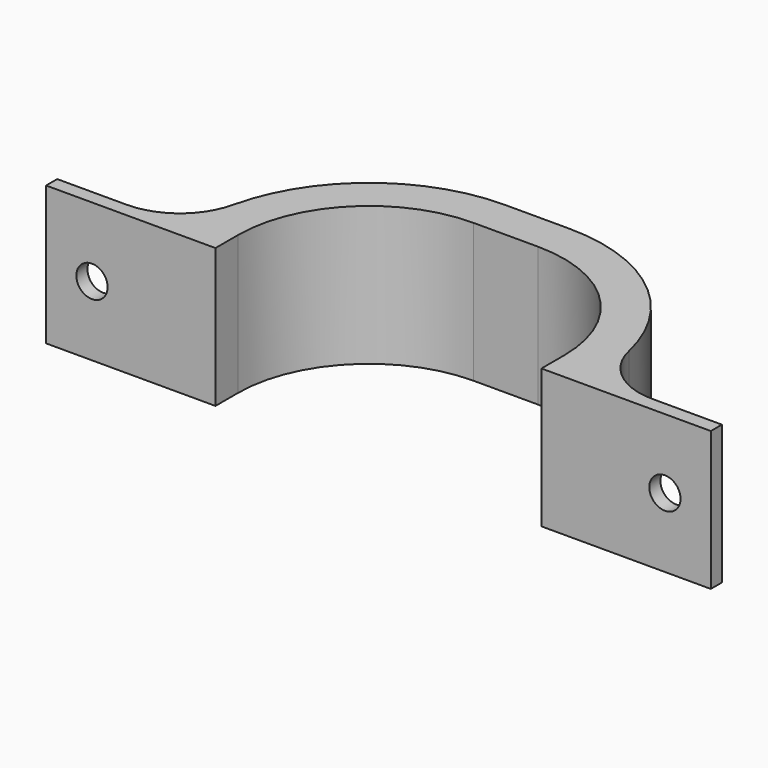
from build123d import *

# Parameters (mm, degrees)
F1_DEPTH = 20
F3_D     = 4.5
F4_D     = 4.5
F5_DEPTH = 2
F6_DEPTH = 2


with BuildPart() as f1:
    # F0 (on Top) → F1 (new body)
    with BuildSketch(Plane.XY):
        with BuildLine():
            Line((-37.8199822518, -7.4723315098), (-45.8199822518, -7.4723315098))
            Line((-45.8199822518, -7.4723315098), (-45.8199822518, -9.4723315098))
            Line((-45.8199822518, -9.4723315098), (-28.8447495745, -9.4723315098))
            Line((-28.8447495745, -9.4723315098), (-23.45, -9.4723315098))
            Line((-23.45, -9.4723315098), (-23.45, -7.887919838))
            Line((-23.45, -7.887919838), (-23.45, -5.3745856304))
            ThreePointArc((-23.45, -5.3745856304), (-17.9429472697, 7.9206157599), (-4.6477458794, 13.4276684902))
            Line((-4.6477458794, 13.4276684902), (0, 13.4276684902))
            Line((0, 13.4276684902), (4.6477458794, 13.4276684902))
            ThreePointArc((4.6477458794, 13.4276684902), (17.9429472697, 7.9206157599), (23.45, -5.3745856304))
            Line((23.45, -5.3745856304), (23.45, -7.887919838))
            Line((23.45, -7.887919838), (23.45, -9.4723315098))
            Line((23.45, -9.4723315098), (28.8447495745, -9.4723315098))
            Line((28.8447495745, -9.4723315098), (45.8199822518, -9.4723315098))
            Line((45.8199822518, -9.4723315098), (45.8199822518, -7.4723315098))
            Line((45.8199822518, -7.4723315098), (37.8199822518, -7.4723315098))
            ThreePointArc((37.8199822518, -7.4723315098), (31.8371692612, -5.3745856304), (28.4743700766, 0))
            ThreePointArc((28.4743700766, 0), (19.9009167747, 13.7024940459), (4.6477458794, 19.0506920822))
            Line((4.6477458794, 19.0506920822), (0, 19.0506920822))
            Line((0, 19.0506920822), (-4.6477458794, 19.0506920822))
            ThreePointArc((-4.6477458794, 19.0506920822), (-19.9009167747, 13.7024940459), (-28.4743700766, 0))
            ThreePointArc((-28.4743700766, 0), (-31.8371692612, -5.3745856304), (-37.8199822518, -7.4723315098))
        make_face()
    extrude(amount=F1_DEPTH)

    # F3 (through all)
    with Locations(Plane(origin=(0, -7.4723315098, 0), x_dir=(-1, 0, 0), z_dir=(0, 1, 0))):
        with Locations((-41.2173499218, 10)):
            Hole(F3_D / 2)

    # F4 (through all)
    with Locations(Plane(origin=(0, -7.4723315098, 0), x_dir=(-1, 0, 0), z_dir=(0, 1, 0))):
        with Locations((41.2173499218, 10)):
            Hole(F4_D / 2)

    # F5 (add): a face of the model
    f5_faces = [f1.faces().sort_by_distance(p)[0] for p in [
        (-45.8199822518, -8.4723315098, 10),
    ]]
    extrude(f5_faces, amount=F5_DEPTH)

    # F6 (add): a face of the model
    f6_faces = [f1.faces().sort_by_distance(p)[0] for p in [
        (45.8199822518, -8.4723315098, 10),
    ]]
    extrude(f6_faces, amount=F6_DEPTH)


solid = f1.part
